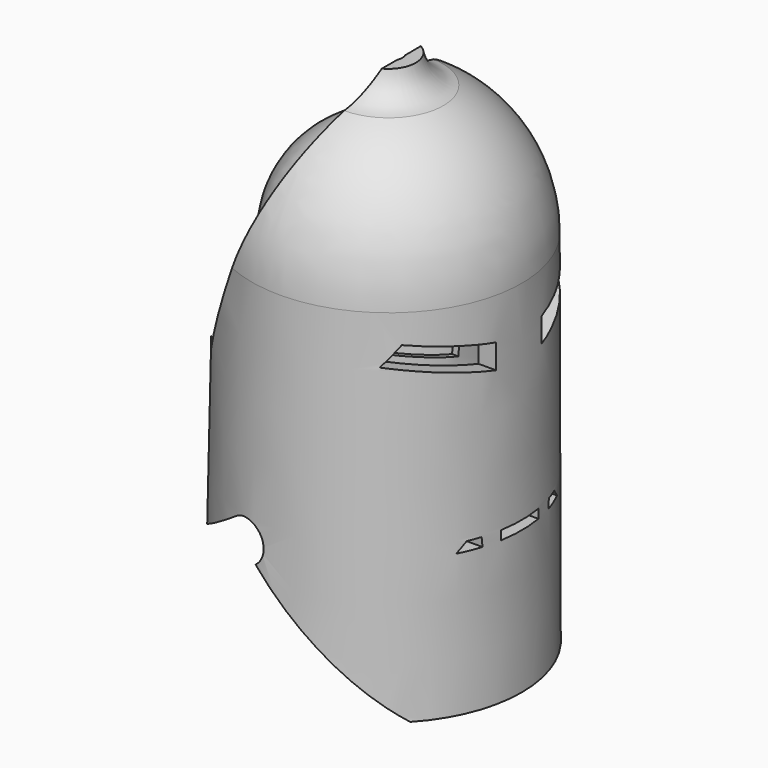
from build123d import *

# Parameters (mm, degrees)
F2_T          = -2.54
F3_ANGLE_BACK = 135
F3_ANGLE      = 270
F6_DEPTH      = 141.478
F7_DEPTH      = 136.8553929726
F10_DEPTH     = 113.538
F11_W         = 9.5853181556
F11_H         = 3.7172362208
F12_DEPTH     = 82.296


# Not quite as in the source:
# - a feature names something its author has since deleted; it is built from what else it names


with BuildPart() as f1:
    # F0 (on Front) → F1 (revolve)
    with BuildSketch(Plane.XZ):
        with BuildLine():
            ThreePointArc((1.4622360468, 80.9415243566), (-28.272207527, 68.6251145587), (-40.5886173248, 38.890670985))
            Line((-40.5886173248, 38.890670985), (-40.5886173248, -55.1905855536))
            Line((-40.5886173248, -55.1905855536), (0, -55.1905855536))
            Line((0, -55.1905855536), (1.4622360468, 80.9415243566))
        make_face()
    revolve(axis=Axis((0.7311180234, 0, 12.8754694015), (-0.010740682, 0, -0.9999423172)))

    # F2
    f2_openings = [f1.faces().sort_by_distance(p)[0] for p in [
        (20.289626, 0, -55.62651),
    ]]
    offset(amount=F2_T, openings=f2_openings)


with BuildPart() as f3:
    # F0 (on Front) → F3 (revolve)
    with BuildSketch(Plane.XZ, mode=Mode.PRIVATE) as f3_sk:
        with BuildLine():
            ThreePointArc((7.6617361046, 88.8827368617), (38.0827744322, 71.7047678623), (50.0726550817, 38.890670985))
            Line((50.0726550817, 38.890670985), (49.6412643201, -109.7343179238))
            Line((49.6412643201, -109.7343179238), (57.0238452832, -109.7343179238))
            Line((57.0238452832, -109.7343179238), (57.0238452832, 38.890670985))
            ThreePointArc((57.0238452832, 38.890670985), (48.2977286312, 70.3711791697), (24.609901011, 92.8668305278))
            ThreePointArc((24.609901011, 92.8668305278), (17.1024457277, 97.0744654518), (13.2324611768, 104.7614216805))
            Line((13.2324611768, 104.7614216805), (7.6617361046, 104.7614216805))
            Line((7.6617361046, 104.7614216805), (7.6617361046, 88.8827368617))
        make_face()
    revolve(f3_sk.sketch.rotate(Axis((0.7311180234, 0, 12.8754694015), (-0.010740682, 0, -0.9999423172)), -F3_ANGLE_BACK), axis=Axis((0.7311180234, 0, 12.8754694015), (-0.010740682, 0, -0.9999423172)), revolution_arc=F3_ANGLE)

    # F5 (on offset) → F6 (cut)
    with BuildSketch(Plane.XZ.offset(79.248)):
        Polygon((-39.1796715558, 0), (7.3632323183, 104.9768552184), (-35.9071232378, 104.9768552184), (-39.1796715558, 104.9768552184), align=None)
    extrude(amount=-F6_DEPTH, mode=Mode.SUBTRACT)


with BuildPart() as f7_tool:
    # F5 (on offset) → F7 (new body, through all)
    with BuildSketch(Plane.XZ.offset(79.248)):
        with BuildLine():
            Line((-17.0782764223, -47.5746723047), (-40.5915752053, -63.8383775949))
            Line((-40.5915752053, -63.8383775949), (-46.4850105345, -67.4691423774))
            Line((-46.4850105345, -67.4691423774), (-46.4850105345, -109.5825880766))
            Line((-46.4850105345, -109.5825880766), (42.0325770974, -109.5825880766))
            Line((42.0325770974, -109.5825880766), (-7.6049312989, -61.270788312))
            ThreePointArc((-7.6049312989, -61.270788312), (-5.493545857, -49.6860577466), (-17.0782764223, -47.5746723047))
        make_face()
    extrude(amount=-F7_DEPTH)


with BuildPart() as f1_1:
    add(f1.part)

    # F7: cut by f7_tool
    add(f7_tool.part, mode=Mode.SUBTRACT)


with BuildPart() as f3_1:
    add(f3.part)

    # F7: cut by f7_tool
    add(f7_tool.part, mode=Mode.SUBTRACT)


with BuildPart() as f10_tool:
    # F9 (on offset) → F10 (new body)
    with BuildSketch(Plane.YZ.offset(93.218)):
        Polygon((11.7156300694, 21.7913519591), (11.7156300694, 11.6589153185), (45.0682379305, 19.2582439631), (40.4242016375, 27.2797569633), align=None)
        Polygon((-11.7156300694, 21.7913519591), (-40.4242016375, 27.2797569633), (-45.0682379305, 19.2582439631), (-11.7156300694, 11.6589153185), align=None)
    extrude(amount=-F10_DEPTH)


with BuildPart() as f1_2:
    add(f1_1.part)

    # F10: cut by f10_tool
    add(f10_tool.part, mode=Mode.SUBTRACT)


with BuildPart() as f3_2:
    add(f3_1.part)

    # F10: cut by f10_tool
    add(f10_tool.part, mode=Mode.SUBTRACT)


with BuildPart() as f12_tool:
    # F11 (on offset) → F12 (new body)
    with BuildSketch(Plane.YZ.offset(93.218)):
        Polygon((-17.0197933912, -50.8276000619), (-17.3295624554, -47.1103638411), (-22.5956495851, -47.1103638411), (-26.0031167418, -50.8276000619), align=None)
        with Locations((4.7926590778, -48.9689819515)):
            Rectangle(F11_W, F11_H)
        with Locations((-4.7926590778, -48.9689819515)):
            Rectangle(F11_W, F11_H)
        Polygon((17.3295624554, -47.1103638411), (17.0197933912, -50.8276000619), (26.0031167418, -50.8276000619), (22.5956495851, -47.1103638411), align=None)
    extrude(amount=-F12_DEPTH)


with BuildPart() as f1_3:
    add(f1_2.part)

    # F12: cut by f12_tool
    add(f12_tool.part, mode=Mode.SUBTRACT)


with BuildPart() as f3_3:
    add(f3_2.part)

    # F12: cut by f12_tool
    add(f12_tool.part, mode=Mode.SUBTRACT)


solid = Compound([f1_3.part, f3_3.part])
